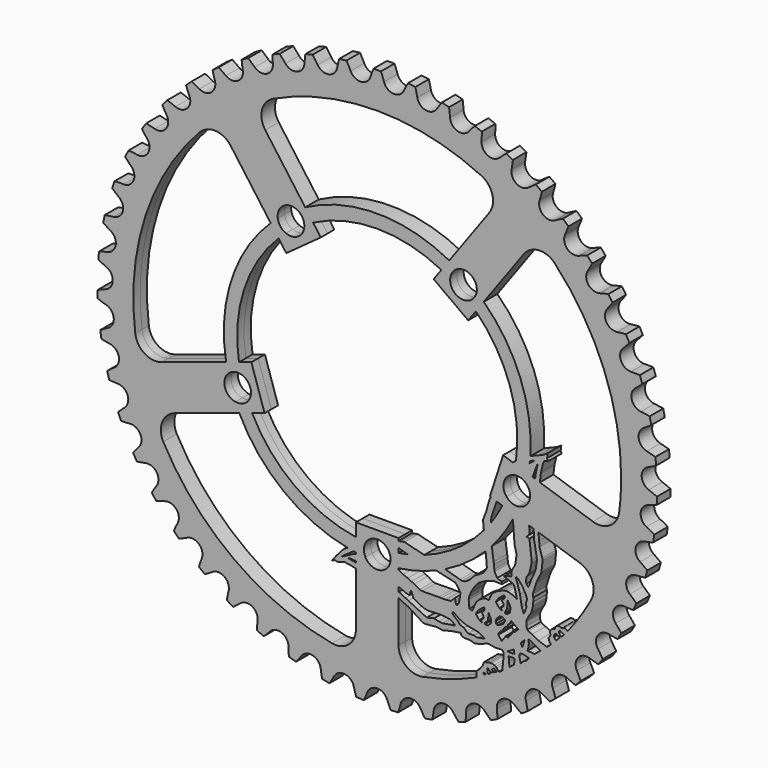
from build123d import *

# Parameters (mm, degrees)
F0_R     = 95.23914061
F2_DEPTH = 3.175
F3_DEPTH = 3.175


# Not quite as in the source:
# - a length typed as a fraction of an inch, garbled in the dataset ("3 / 203.2 mm" for 3/8 in), is restored


with BuildPart() as f2:
    # F0 (on Front) → F2 (new body, symmetric)
    with BuildSketch(Plane.XZ):
        with BuildLine():
            ThreePointArc((1.3974512393, 104.8471286678), (0, 104.8564411939), (-1.3974512393, 104.8471286678))
            ThreePointArc((-1.3974512393, 104.8471286678), (-1.9989055088, 103.3019703404), (-2.5462079028, 101.7368116953))
            ThreePointArc((-2.5462079028, 101.7368116953), (-3.9052398194, 99.8191421504), (-6.1056801538, 98.9930146972))
            ThreePointArc((-6.1056801538, 98.9930146972), (-8.3909636625, 99.5424721739), (-9.9753539423, 101.2785976519))
            ThreePointArc((-9.9753539423, 101.2785976519), (-10.7108477336, 102.7646361365), (-11.4976251519, 104.2241712642))
            ThreePointArc((-11.4976251519, 104.2241712642), (-12.8856288235, 104.061682812), (-14.2713436942, 103.880710476))
            ThreePointArc((-14.2713436942, 103.880710476), (-14.6783573813, 102.2733519742), (-15.0291718315, 100.6527993782))
            ThreePointArc((-15.0291718315, 100.6527993782), (-16.1422438465, 98.5826556819), (-18.224484574, 97.4923815023))
            ThreePointArc((-18.224484574, 97.4923815023), (-20.5599686886, 97.7568397874), (-22.34569959, 99.2851033058))
            ThreePointArc((-22.34569959, 99.2851033058), (-23.2582354424, 100.6694948013), (-24.2184092659, 102.0212816645))
            ThreePointArc((-24.2184092659, 102.0212816645), (-25.5759246489, 101.6894553933), (-26.9288971262, 101.3395666036))
            ThreePointArc((-26.9288971262, 101.3395666036), (-27.1353003181, 99.6943738437), (-27.2843088352, 98.0429932223))
            ThreePointArc((-27.2843088352, 98.0429932223), (-28.1345479113, 95.8517566428), (-30.0670243851, 94.5138631821))
            ThreePointArc((-30.0670243851, 94.5138631821), (-32.417305547, 94.4893133574), (-34.3773072098, 95.7865479992))
            ThreePointArc((-34.3773072098, 95.7865479992), (-35.45305201, 97.0483065417), (-36.5720669823, 98.2718534296))
            ThreePointArc((-36.5720669823, 98.2718534296), (-37.8785155273, 97.7757194874), (-39.1782359275, 97.2622182014))
            ThreePointArc((-39.1782359275, 97.2622182014), (-39.1808997623, 95.6041306286), (-39.125843529, 93.9469552287))
            ThreePointArc((-39.125843529, 93.9469552287), (-39.7003609085, 91.667842679), (-41.4537787551, 90.1026110382))
            ThreePointArc((-41.4537787551, 90.1026110382), (-43.7832290977, 89.7894252541), (-45.8877898946, 90.8359662645))
            ThreePointArc((-45.8877898946, 90.8359662645), (-47.110436448, 91.9559648806), (-48.3713294427, 93.0327240695))
            ThreePointArc((-48.3713294427, 93.0327240695), (-49.6069067216, 92.3798033412), (-50.8336726082, 91.7104737148))
            ThreePointArc((-50.8336726082, 91.7104737148), (-50.632556705, 90.0646262467), (-50.3742703176, 88.4267771581))
            ThreePointArc((-50.3742703176, 88.4267771581), (-50.6643569028, 86.0943376612), (-52.2121360949, 84.3254951565))
            ThreePointArc((-52.2121360949, 84.3254951565), (-54.4854435255, 83.7284209902), (-56.70266046, 84.5084038742))
            ThreePointArc((-56.70266046, 84.5084038742), (-58.0536746912, 85.4696645266), (-59.4373318558, 86.3833134448))
            ThreePointArc((-59.4373318558, 86.3833134448), (-60.5833077764, 85.5835035431), (-61.7185226292, 84.7684919313))
            ThreePointArc((-61.7185226292, 84.7684919313), (-61.3166757, 83.1598339377), (-60.8590745169, 81.5661392831))
            ThreePointArc((-60.8590745169, 81.5661392831), (-60.8603328907, 79.2157302442), (-62.1790106736, 77.2700907249))
            ThreePointArc((-62.1790106736, 77.2700907249), (-64.3617141688, 76.3981792122), (-66.6579764924, 76.8997802243))
            ThreePointArc((-66.6579764924, 76.8997802243), (-68.1168784028, 77.6877311814), (-69.6023249051, 78.4244198426))
            ThreePointArc((-69.6023249051, 78.4244198426), (-70.6413276406, 77.4898450703), (-71.6677827595, 76.5415062183))
            ThreePointArc((-71.6677827595, 76.5415062183), (-71.0712963941, 74.9944233147), (-70.4213171828, 73.4690418805))
            ThreePointArc((-70.4213171828, 73.4690418805), (-70.1337282697, 71.1362931047), (-71.2033148323, 69.0433504827))
            ThreePointArc((-71.2033148323, 69.0433504827), (-73.2623268321, 67.9098189133), (-75.6028255485, 68.1254342936))
            ThreePointArc((-75.6028255485, 68.1254342936), (-77.1474996722, 68.7281310219), (-78.7122176575, 69.276691977))
            ThreePointArc((-78.7122176575, 69.276691977), (-79.6284969855, 68.221519535), (-80.5306323574, 67.1542292932))
            ThreePointArc((-80.5306323574, 67.1542292932), (-79.748548681, 65.6921736793), (-78.9160444638, 64.2582286932))
            ThreePointArc((-78.9160444638, 64.2582286932), (-78.3439678185, 61.9785022741), (-79.1482493188, 59.7699834261))
            ThreePointArc((-79.1482493188, 59.7699834261), (-81.0523573, 58.3920149832), (-83.4016128346, 58.3183762222))
            ThreePointArc((-83.4016128346, 58.3183762222), (-85.0086434865, 58.7266824538), (-86.628913425, 59.0788000779))
            ThreePointArc((-86.628913425, 59.0788000779), (-87.408579485, 57.9190253048), (-88.172719657, 56.7489627052))
            ThreePointArc((-88.172719657, 56.7489627052), (-87.2168942611, 55.3940976539), (-86.2144849533, 54.0733262601))
            ThreePointArc((-86.2144849533, 54.0733262601), (-85.3665926745, 51.8811805265), (-85.8933770249, 49.5905643469))
            ThreePointArc((-85.8933770249, 49.5905643469), (-87.6137166516, 47.9890476274), (-89.9361166851, 47.6272710137))
            ThreePointArc((-89.9361166851, 47.6272710137), (-91.5811429185, 47.8349972424), (-93.2324031697, 47.9853337911))
            ThreePointArc((-93.2324031697, 47.9853337911), (-93.8636370189, 46.7385376903), (-94.478198405, 45.4834396894))
            ThreePointArc((-94.478198405, 45.4834396894), (-93.3631206282, 44.2563035737), (-92.2060017332, 43.0687273203))
            ThreePointArc((-92.2060017332, 43.0687273203), (-91.0951470036, 40.9973929669), (-91.3364486902, 38.6594028621))
            ThreePointArc((-91.3364486902, 38.6594028621), (-92.8469413671, 36.858615227), (-95.1072806824, 36.2141849253))
            ThreePointArc((-95.1072806824, 36.2141849253), (-96.7653655766, 36.2181822331), (-98.4225847182, 36.1644587577))
            ThreePointArc((-98.4225847182, 36.1644587577), (-98.8958174949, 34.8495414871), (-99.351483971, 33.5284340911))
            ThreePointArc((-99.351483971, 33.5284340911), (-98.0940572557, 32.4476290436), (-96.7997695163, 31.4112503761))
            ThreePointArc((-96.7997695163, 31.4112503761), (-95.4427917614, 29.4921267203), (-95.3949528966, 27.1422042371))
            ThreePointArc((-95.3949528966, 27.1422042371), (-96.6727010946, 25.1694437913), (-98.8367152516, 24.252128708))
            ThreePointArc((-98.8367152516, 24.252128708), (-100.4827239298, 24.0523364999), (-102.1207802088, 23.7953673935))
            ThreePointArc((-102.1207802088, 23.7953673935), (-102.4288381865, 22.4322617587), (-102.7187023133, 21.065171609))
            ThreePointArc((-102.7187023133, 21.065171609), (-101.3379879668, 20.1470815326), (-99.9261514659, 19.2776108951))
            ThreePointArc((-99.9261514659, 19.2776108951), (-98.343621085, 17.5397898952), (-98.0073668573, 15.2135574631))
            ThreePointArc((-98.0073668573, 15.2135574631), (-99.0330012161, 13.0987292441), (-101.0678859662, 11.9224349409))
            ThreePointArc((-101.0678859662, 11.9224349409), (-102.6768666145, 11.5218818629), (-104.2709287676, 11.0655625153))
            ThreePointArc((-104.2709287676, 11.0655625153), (-104.4091421014, 9.6749318081), (-104.5288098342, 8.2825825979))
            ThreePointArc((-104.5288098342, 8.2825825979), (-103.0457380786, 7.5411248023), (-101.5377548183, 6.8517424834))
            ThreePointArc((-101.5377548183, 6.8517424834), (-99.753661359, 5.3215677344), (-99.1340890397, 3.0542886658))
            ThreePointArc((-99.1340890397, 3.0542886658), (-99.8920619879, 0.8294513136), (-101.7669705525, -0.5879907869))
            ThreePointArc((-101.7669705525, -0.5879907869), (-103.3145326645, -1.1832327583), (-104.8404363343, -1.831985011))
            ThreePointArc((-104.8404363343, -1.831985011), (-104.8067098509, -3.2290602466), (-104.7543671488, -4.6255619225))
            ThreePointArc((-104.7543671488, -4.6255619225), (-103.1914198401, -5.1791476929), (-101.6101493096, -5.67799136))
            ThreePointArc((-101.6101493096, -5.67799136), (-99.6515378101, -6.9773239687), (-98.758039484, -9.1512800343))
            ThreePointArc((-98.758039484, -9.1512800343), (-99.2368609244, -11.4524002533), (-100.9233716008, -13.0895031738))
            ThreePointArc((-100.9233716008, -13.0895031738), (-102.3860557123, -13.870410777), (-103.8206697546, -14.701761512))
            ThreePointArc((-103.8206697546, -14.701761512), (-103.6155147131, -16.0841030394), (-103.3919550381, -17.4635876392))
            ThreePointArc((-103.3919550381, -17.4635876392), (-101.7728248644, -17.8209095885), (-100.142237513, -18.1216526423))
            ThreePointArc((-100.142237513, -18.1216526423), (-98.0387985272, -19.1704465528), (-96.8849187181, -21.2181246574))
            ThreePointArc((-96.8849187181, -21.2181246574), (-97.0773302057, -23.5606451062), (-98.5498772112, -25.3925920352))
            ThreePointArc((-98.5498772112, -25.3925920352), (-99.9055105221, -26.3473275071), (-101.2270876503, -27.3486742946))
            ThreePointArc((-101.2270876503, -27.3486742946), (-100.8536139921, -28.6953272254), (-100.4622262811, -30.0368831687))
            ThreePointArc((-100.4622262811, -30.0368831687), (-98.8114576053, -30.1925246603), (-97.1562714752, -30.2906081427))
            ThreePointArc((-97.1562714752, -30.2906081427), (-94.9398909938, -31.0729647084), (-93.5431213435, -32.9633241392))
            ThreePointArc((-93.5431213435, -32.9633241392), (-93.4462061162, -35.3117345958), (-94.6824671393, -37.3107550852))
            ThreePointArc((-94.6824671393, -37.3107550852), (-95.9104996304, -38.4248456091), (-97.0990060825, -39.5810090527))
            ThreePointArc((-97.0990060825, -39.5810090527), (-96.5628752875, -40.8715595011), (-96.0095925791, -42.1548501673))
            ThreePointArc((-96.0095925791, -42.1548501673), (-94.3522093717, -42.1064518349), (-92.6975153974, -42.0003889001))
            ThreePointArc((-92.6975153974, -42.0003889001), (-90.4017914894, -42.504448393), (-88.7833056019, -44.2088332281))
            ThreePointArc((-88.7833056019, -44.2088332281), (-88.3985327959, -46.5275341837), (-89.3797673795, -48.6633251205))
            ThreePointArc((-89.3797673795, -48.6633251205), (-90.4615833302, -49.9198822198), (-91.4990025598, -51.2133360601))
            ThreePointArc((-91.4990025598, -51.2133360601), (-90.8083418243, -52.4282205969), (-90.1015513205, -53.6337926077))
            ThreePointArc((-90.1015513205, -53.6337926077), (-88.4626778214, -53.3820881206), (-86.8335594768, -53.0734865747))
            ThreePointArc((-86.8335594768, -53.0734865747), (-84.4932929765, -53.2916079667), (-82.6776254481, -54.7841814692))
            ThreePointArc((-82.6776254481, -54.7841814692), (-82.0108278269, -57.0380237809), (-82.722161455, -59.2782087517))
            ThreePointArc((-82.722161455, -59.2782087517), (-83.6413616381, -60.6581843016), (-84.5119674272, -62.0693210969))
            ThreePointArc((-84.5119674272, -62.0693210969), (-83.677246464, -63.1901233109), (-82.8276623883, -64.2997014234))
            ThreePointArc((-82.8276623883, -64.2997014234), (-81.2321422492, -63.8485063651), (-79.6532953078, -63.342044293))
            ThreePointArc((-79.6532953078, -63.342044293), (-77.3039622698, -63.270921086), (-75.3186367695, -64.5290573631))
            ThreePointArc((-75.3186367695, -64.5290573631), (-74.3799223052, -66.683875079), (-74.8105718852, -68.9944951631))
            ThreePointArc((-74.8105718852, -68.9944951631), (-75.5532221629, -70.476970141), (-76.2438170152, -71.9843984958))
            ThreePointArc((-76.2438170152, -71.9843984958), (-75.2776893432, -72.9941281679), (-74.2981905242, -73.990892309))
            ThreePointArc((-74.2981905242, -73.990892309), (-72.770210204, -73.3470463367), (-71.265568376, -72.6504011871))
            ThreePointArc((-71.265568376, -72.6504011871), (-68.9427822944, -72.2911115366), (-66.817894333, -73.2957385248))
            ThreePointArc((-66.817894333, -73.2957385248), (-65.6214929802, -75.3188668047), (-65.7649303033, -77.664895357))
            ThreePointArc((-65.7649303033, -77.664895357), (-66.3197728544, -79.2273969532), (-66.8198880558, -80.8082657904))
            ThreePointArc((-66.8198880558, -80.8082657904), (-65.7369991858, -81.691616448), (-64.6424338271, -82.5604566893))
            ThreePointArc((-64.6424338271, -82.5604566893), (-63.20515595, -81.7337198516), (-61.7975280718, -80.857452055))
            ThreePointArc((-61.7975280718, -80.857452055), (-59.5365000158, -80.2154424257), (-57.3042607288, -80.9513310039))
            ThreePointArc((-57.3042607288, -80.9513310039), (-55.8683087124, -82.8121012854), (-55.7223594151, -85.1579749044))
            ThreePointArc((-55.7223594151, -85.1579749044), (-56.0809833921, -86.7768171877), (-56.3830377061, -88.407162147))
            ThreePointArc((-56.3830377061, -88.407162147), (-55.1998031293, -89.1507430946), (-54.006763726, -89.8784887038))
            ThreePointArc((-54.006763726, -89.8784887038), (-52.6819759595, -88.8813934884), (-51.3927002349, -87.8387863712))
            ThreePointArc((-51.3927002349, -87.8387863712), (-49.2277050852, -86.9237889748), (-46.9219529448, -87.3797838223))
            ThreePointArc((-46.9219529448, -87.3797838223), (-45.2682178335, -89.0499887246), (-44.8350943583, -91.3601463576))
            ThreePointArc((-44.8350943583, -91.3601463576), (-44.9920633874, -93.0107893289), (-45.0914779783, -94.6658960427))
            ThreePointArc((-45.0914779783, -94.6658960427), (-43.825834325, -95.2584353512), (-42.5524061384, -95.8340544466))
            ThreePointArc((-42.5524061384, -95.8340544466), (-41.3601909146, -94.6817158006), (-40.2088114494, -93.488574224))
            ThreePointArc((-40.2088114494, -93.488574224), (-38.1726683254, -92.3144594882), (-35.8283561837, -92.483648188))
            ThreePointArc((-35.8283561837, -92.483648188), (-33.9819069162, -93.9379691074), (-33.2681749735, -96.1773911194))
            ThreePointArc((-33.2681749735, -96.1773911194), (-33.2211095641, -97.834812714), (-33.1163774082, -99.4895914516))
            ThreePointArc((-33.1163774082, -99.4895914516), (-31.7875105459, -99.9221068289), (-30.4529974492, -100.3368736118))
            ThreePointArc((-30.4529974492, -100.3368736118), (-29.4114275356, -99.0467598146), (-28.4153980688, -97.7211705886))
            ThreePointArc((-28.4153980688, -97.7211705886), (-26.5389728249, -96.305736896), (-24.1916380643, -96.1855547198))
            ThreePointArc((-24.1916380643, -96.1855547198), (-22.1804649293, -97.4019456336), (-21.1969439678, -99.5366846697))
            ThreePointArc((-21.1969439678, -99.5366846697), (-20.9465575835, -101.1757600656), (-20.6392663135, -102.8051260681))
            ThreePointArc((-20.6392663135, -102.8051260681), (-19.2673205093, -103.0710610221), (-17.8919523608, -103.3186880509))
            ThreePointArc((-17.8919523608, -103.3186880509), (-17.0168168956, -101.9103559124), (-16.1912362186, -100.4724136185))
            ThreePointArc((-16.1912362186, -100.4724136185), (-14.5029735487, -98.8371175011), (-12.1881993714, -98.4293862882))
            ThreePointArc((-12.1881993714, -98.4293862882), (-10.0427897036, -99.38940795), (-8.8043888985, -101.3871035425))
            ThreePointArc((-8.8043888985, -101.3871035425), (-8.3544771417, -102.9829860275), (-7.84928498, -104.5622397672))
            ThreePointArc((-7.84928498, -104.5622397672), (-6.4550575339, -104.6575629951), (-5.0596835126, -104.7342964964))
            ThreePointArc((-5.0596835126, -104.7342964964), (-4.3642486574, -103.2290948963), (-3.7216317317, -101.7005972739))
            ThreePointArc((-3.7216317317, -101.7005972739), (-2.247123977, -99.8702281539), (0, -99.1811286939))
            ThreePointArc((0, -99.1811286939), (2.247123977, -99.8702281539), (3.7216317317, -101.7005972739))
            ThreePointArc((3.7216317317, -101.7005972739), (4.3642486574, -103.2290948963), (5.0596835126, -104.7342964964))
            ThreePointArc((5.0596835126, -104.7342964964), (6.4550575339, -104.6575629951), (7.84928498, -104.5622397672))
            ThreePointArc((7.84928498, -104.5622397672), (8.3544771417, -102.9829860275), (8.8043888985, -101.3871035425))
            ThreePointArc((8.8043888985, -101.3871035425), (10.0427897036, -99.38940795), (12.1881993714, -98.4293862882))
            ThreePointArc((12.1881993714, -98.4293862882), (14.5029735487, -98.8371175011), (16.1912362186, -100.4724136185))
            ThreePointArc((16.1912362186, -100.4724136185), (17.0168168956, -101.9103559124), (17.8919523608, -103.3186880509))
            ThreePointArc((17.8919523608, -103.3186880509), (19.2673205093, -103.0710610221), (20.6392663135, -102.8051260681))
            ThreePointArc((20.6392663135, -102.8051260681), (20.9465575835, -101.1757600656), (21.1969439678, -99.5366846697))
            ThreePointArc((21.1969439678, -99.5366846697), (22.1804649293, -97.4019456336), (24.1916380643, -96.1855547198))
            ThreePointArc((24.1916380643, -96.1855547198), (26.5389728249, -96.305736896), (28.4153980688, -97.7211705886))
            ThreePointArc((28.4153980688, -97.7211705886), (29.4114275356, -99.0467598146), (30.4529974492, -100.3368736118))
            ThreePointArc((30.4529974492, -100.3368736118), (31.7875105459, -99.9221068289), (33.1163774082, -99.4895914516))
            ThreePointArc((33.1163774082, -99.4895914516), (33.2211095641, -97.834812714), (33.2681749735, -96.1773911194))
            ThreePointArc((33.2681749735, -96.1773911194), (33.9819069162, -93.9379691074), (35.8283561837, -92.483648188))
            ThreePointArc((35.8283561837, -92.483648188), (38.1726683254, -92.3144594882), (40.2088114494, -93.488574224))
            ThreePointArc((40.2088114494, -93.488574224), (41.3601909146, -94.6817158006), (42.5524061384, -95.8340544466))
            ThreePointArc((42.5524061384, -95.8340544466), (43.825834325, -95.2584353512), (45.0914779783, -94.6658960427))
            ThreePointArc((45.0914779783, -94.6658960427), (44.9920633874, -93.0107893289), (44.8350943583, -91.3601463576))
            ThreePointArc((44.8350943583, -91.3601463576), (45.2682178335, -89.0499887246), (46.9219529448, -87.3797838223))
            ThreePointArc((46.9219529448, -87.3797838223), (49.2277050852, -86.9237889748), (51.3927002349, -87.8387863712))
            ThreePointArc((51.3927002349, -87.8387863712), (52.6819759595, -88.8813934884), (54.006763726, -89.8784887038))
            ThreePointArc((54.006763726, -89.8784887038), (55.1998031293, -89.1507430946), (56.3830377061, -88.407162147))
            ThreePointArc((56.3830377061, -88.407162147), (56.0809833921, -86.7768171877), (55.7223594151, -85.1579749044))
            ThreePointArc((55.7223594151, -85.1579749044), (55.8683087124, -82.8121012854), (57.3042607288, -80.9513310039))
            ThreePointArc((57.3042607288, -80.9513310039), (59.5365000158, -80.2154424257), (61.7975280718, -80.857452055))
            ThreePointArc((61.7975280718, -80.857452055), (63.20515595, -81.7337198516), (64.6424338271, -82.5604566893))
            ThreePointArc((64.6424338271, -82.5604566893), (65.7369991858, -81.691616448), (66.8198880558, -80.8082657904))
            ThreePointArc((66.8198880558, -80.8082657904), (66.3197728544, -79.2273969532), (65.7649303033, -77.664895357))
            ThreePointArc((65.7649303033, -77.664895357), (65.6214929802, -75.3188668047), (66.817894333, -73.2957385248))
            ThreePointArc((66.817894333, -73.2957385248), (68.9427822944, -72.2911115366), (71.265568376, -72.6504011871))
            ThreePointArc((71.265568376, -72.6504011871), (72.770210204, -73.3470463367), (74.2981905242, -73.990892309))
            ThreePointArc((74.2981905242, -73.990892309), (75.2776893432, -72.9941281679), (76.2438170152, -71.9843984958))
            ThreePointArc((76.2438170152, -71.9843984958), (75.5532221629, -70.476970141), (74.8105718852, -68.9944951631))
            ThreePointArc((74.8105718852, -68.9944951631), (74.3799223052, -66.683875079), (75.3186367695, -64.5290573631))
            ThreePointArc((75.3186367695, -64.5290573631), (77.3039622698, -63.270921086), (79.6532953078, -63.342044293))
            ThreePointArc((79.6532953078, -63.342044293), (81.2321422492, -63.8485063651), (82.8276623883, -64.2997014234))
            ThreePointArc((82.8276623883, -64.2997014234), (83.677246464, -63.1901233109), (84.5119674272, -62.0693210969))
            ThreePointArc((84.5119674272, -62.0693210969), (83.6413616381, -60.6581843016), (82.722161455, -59.2782087517))
            ThreePointArc((82.722161455, -59.2782087517), (82.0108278269, -57.0380237809), (82.6776254481, -54.7841814692))
            ThreePointArc((82.6776254481, -54.7841814692), (84.4932929765, -53.2916079667), (86.8335594768, -53.0734865747))
            ThreePointArc((86.8335594768, -53.0734865747), (88.4626778214, -53.3820881206), (90.1015513205, -53.6337926077))
            ThreePointArc((90.1015513205, -53.6337926077), (90.8083418243, -52.4282205969), (91.4990025598, -51.2133360601))
            ThreePointArc((91.4990025598, -51.2133360601), (90.4615833302, -49.9198822198), (89.3797673795, -48.6633251205))
            ThreePointArc((89.3797673795, -48.6633251205), (88.3985327959, -46.5275341837), (88.7833056019, -44.2088332281))
            ThreePointArc((88.7833056019, -44.2088332281), (90.4017914894, -42.504448393), (92.6975153974, -42.0003889001))
            ThreePointArc((92.6975153974, -42.0003889001), (94.3522093717, -42.1064518349), (96.0095925791, -42.1548501673))
            ThreePointArc((96.0095925791, -42.1548501673), (96.5628752875, -40.8715595011), (97.0990060825, -39.5810090527))
            ThreePointArc((97.0990060825, -39.5810090527), (95.9104996304, -38.4248456091), (94.6824671393, -37.3107550852))
            ThreePointArc((94.6824671393, -37.3107550852), (93.4462061162, -35.3117345958), (93.5431213435, -32.9633241392))
            ThreePointArc((93.5431213435, -32.9633241392), (94.9398909938, -31.0729647084), (97.1562714752, -30.2906081427))
            ThreePointArc((97.1562714752, -30.2906081427), (98.8114576053, -30.1925246603), (100.4622262811, -30.0368831687))
            ThreePointArc((100.4622262811, -30.0368831687), (100.8536139921, -28.6953272254), (101.2270876503, -27.3486742946))
            ThreePointArc((101.2270876503, -27.3486742946), (99.9055105221, -26.3473275071), (98.5498772112, -25.3925920352))
            ThreePointArc((98.5498772112, -25.3925920352), (97.0773302057, -23.5606451062), (96.8849187181, -21.2181246574))
            ThreePointArc((96.8849187181, -21.2181246574), (98.0387985272, -19.1704465528), (100.142237513, -18.1216526423))
            ThreePointArc((100.142237513, -18.1216526423), (101.7728248644, -17.8209095885), (103.3919550381, -17.4635876392))
            ThreePointArc((103.3919550381, -17.4635876392), (103.6155147131, -16.0841030394), (103.8206697546, -14.701761512))
            ThreePointArc((103.8206697546, -14.701761512), (102.3860557123, -13.870410777), (100.9233716008, -13.0895031738))
            ThreePointArc((100.9233716008, -13.0895031738), (99.2368609244, -11.4524002533), (98.758039484, -9.1512800343))
            ThreePointArc((98.758039484, -9.1512800343), (99.6515378101, -6.9773239687), (101.6101493096, -5.67799136))
            ThreePointArc((101.6101493096, -5.67799136), (103.1914198401, -5.1791476929), (104.7543671488, -4.6255619225))
            ThreePointArc((104.7543671488, -4.6255619225), (104.8067098509, -3.2290602466), (104.8404363343, -1.831985011))
            ThreePointArc((104.8404363343, -1.831985011), (103.3145326645, -1.1832327583), (101.7669705525, -0.5879907869))
            ThreePointArc((101.7669705525, -0.5879907869), (99.8920619879, 0.8294513136), (99.1340890397, 3.0542886658))
            ThreePointArc((99.1340890397, 3.0542886658), (99.753661359, 5.3215677344), (101.5377548183, 6.8517424834))
            ThreePointArc((101.5377548183, 6.8517424834), (103.0457380786, 7.5411248023), (104.5288098342, 8.2825825979))
            ThreePointArc((104.5288098342, 8.2825825979), (104.4091421014, 9.6749318081), (104.2709287676, 11.0655625153))
            ThreePointArc((104.2709287676, 11.0655625153), (102.6768666145, 11.5218818629), (101.0678859662, 11.9224349409))
            ThreePointArc((101.0678859662, 11.9224349409), (99.0330012161, 13.0987292441), (98.0073668573, 15.2135574631))
            ThreePointArc((98.0073668573, 15.2135574631), (98.343621085, 17.5397898952), (99.9261514659, 19.2776108951))
            ThreePointArc((99.9261514659, 19.2776108951), (101.3379879668, 20.1470815326), (102.7187023133, 21.065171609))
            ThreePointArc((102.7187023133, 21.065171609), (102.4288381865, 22.4322617587), (102.1207802088, 23.7953673935))
            ThreePointArc((102.1207802088, 23.7953673935), (100.4827239298, 24.0523364999), (98.8367152516, 24.252128708))
            ThreePointArc((98.8367152516, 24.252128708), (96.6727010946, 25.1694437913), (95.3949528966, 27.1422042371))
            ThreePointArc((95.3949528966, 27.1422042371), (95.4427917614, 29.4921267203), (96.7997695163, 31.4112503761))
            ThreePointArc((96.7997695163, 31.4112503761), (98.0940572557, 32.4476290436), (99.351483971, 33.5284340911))
            ThreePointArc((99.351483971, 33.5284340911), (98.8958174949, 34.8495414871), (98.4225847182, 36.1644587577))
            ThreePointArc((98.4225847182, 36.1644587577), (96.7653655766, 36.2181822331), (95.1072806824, 36.2141849253))
            ThreePointArc((95.1072806824, 36.2141849253), (92.8469413671, 36.858615227), (91.3364486902, 38.6594028621))
            ThreePointArc((91.3364486902, 38.6594028621), (91.0951470036, 40.9973929669), (92.2060017332, 43.0687273203))
            ThreePointArc((92.2060017332, 43.0687273203), (93.3631206282, 44.2563035737), (94.478198405, 45.4834396894))
            ThreePointArc((94.478198405, 45.4834396894), (93.8636370189, 46.7385376903), (93.2324031697, 47.9853337911))
            ThreePointArc((93.2324031697, 47.9853337911), (91.5811429185, 47.8349972424), (89.9361166851, 47.6272710137))
            ThreePointArc((89.9361166851, 47.6272710137), (87.6137166516, 47.9890476274), (85.8933770249, 49.5905643469))
            ThreePointArc((85.8933770249, 49.5905643469), (85.3665926745, 51.8811805265), (86.2144849533, 54.0733262601))
            ThreePointArc((86.2144849533, 54.0733262601), (87.2168942611, 55.3940976539), (88.172719657, 56.7489627052))
            ThreePointArc((88.172719657, 56.7489627052), (87.408579485, 57.9190253048), (86.628913425, 59.0788000779))
            ThreePointArc((86.628913425, 59.0788000779), (85.0086434865, 58.7266824538), (83.4016128346, 58.3183762222))
            ThreePointArc((83.4016128346, 58.3183762222), (81.0523573, 58.3920149832), (79.1482493188, 59.7699834261))
            ThreePointArc((79.1482493188, 59.7699834261), (78.3439678185, 61.9785022741), (78.9160444638, 64.2582286932))
            ThreePointArc((78.9160444638, 64.2582286932), (79.748548681, 65.6921736793), (80.5306323574, 67.1542292932))
            ThreePointArc((80.5306323574, 67.1542292932), (79.6284969855, 68.221519535), (78.7122176575, 69.276691977))
            ThreePointArc((78.7122176575, 69.276691977), (77.1474996722, 68.7281310219), (75.6028255485, 68.1254342936))
            ThreePointArc((75.6028255485, 68.1254342936), (73.2623268321, 67.9098189133), (71.2033148323, 69.0433504827))
            ThreePointArc((71.2033148323, 69.0433504827), (70.1337282697, 71.1362931047), (70.4213171828, 73.4690418805))
            ThreePointArc((70.4213171828, 73.4690418805), (71.0712963941, 74.9944233147), (71.6677827595, 76.5415062183))
            ThreePointArc((71.6677827595, 76.5415062183), (70.6413276406, 77.4898450703), (69.6023249051, 78.4244198426))
            ThreePointArc((69.6023249051, 78.4244198426), (68.1168784028, 77.6877311814), (66.6579764924, 76.8997802243))
            ThreePointArc((66.6579764924, 76.8997802243), (64.3617141688, 76.3981792122), (62.1790106736, 77.2700907249))
            ThreePointArc((62.1790106736, 77.2700907249), (60.8603328907, 79.2157302442), (60.8590745169, 81.5661392831))
            ThreePointArc((60.8590745169, 81.5661392831), (61.3166757, 83.1598339377), (61.7185226292, 84.7684919313))
            ThreePointArc((61.7185226292, 84.7684919313), (60.5833077764, 85.5835035431), (59.4373318558, 86.3833134448))
            ThreePointArc((59.4373318558, 86.3833134448), (58.0536746912, 85.4696645266), (56.70266046, 84.5084038742))
            ThreePointArc((56.70266046, 84.5084038742), (54.4854435255, 83.7284209902), (52.2121360949, 84.3254951565))
            ThreePointArc((52.2121360949, 84.3254951565), (50.6643569028, 86.0943376612), (50.3742703176, 88.4267771581))
            ThreePointArc((50.3742703176, 88.4267771581), (50.632556705, 90.0646262467), (50.8336726082, 91.7104737148))
            ThreePointArc((50.8336726082, 91.7104737148), (49.6069067216, 92.3798033412), (48.3713294427, 93.0327240695))
            ThreePointArc((48.3713294427, 93.0327240695), (47.110436448, 91.9559648806), (45.8877898946, 90.8359662645))
            ThreePointArc((45.8877898946, 90.8359662645), (43.7832290977, 89.7894252541), (41.4537787551, 90.1026110382))
            ThreePointArc((41.4537787551, 90.1026110382), (39.7003609085, 91.667842679), (39.125843529, 93.9469552287))
            ThreePointArc((39.125843529, 93.9469552287), (39.1808997623, 95.6041306286), (39.1782359275, 97.2622182014))
            ThreePointArc((39.1782359275, 97.2622182014), (37.8785155273, 97.7757194874), (36.5720669823, 98.2718534296))
            ThreePointArc((36.5720669823, 98.2718534296), (35.45305201, 97.0483065417), (34.3773072098, 95.7865479992))
            ThreePointArc((34.3773072098, 95.7865479992), (32.417305547, 94.4893133574), (30.0670243851, 94.5138631821))
            ThreePointArc((30.0670243851, 94.5138631821), (28.1345479113, 95.8517566428), (27.2843088352, 98.0429932223))
            ThreePointArc((27.2843088352, 98.0429932223), (27.1353003181, 99.6943738437), (26.9288971262, 101.3395666036))
            ThreePointArc((26.9288971262, 101.3395666036), (25.5759246489, 101.6894553933), (24.2184092659, 102.0212816645))
            ThreePointArc((24.2184092659, 102.0212816645), (23.2582354424, 100.6694948013), (22.34569959, 99.2851033058))
            ThreePointArc((22.34569959, 99.2851033058), (20.5599686886, 97.7568397874), (18.224484574, 97.4923815023))
            ThreePointArc((18.224484574, 97.4923815023), (16.1422438465, 98.5826556819), (15.0291718315, 100.6527993782))
            ThreePointArc((15.0291718315, 100.6527993782), (14.6783573813, 102.2733519742), (14.2713436942, 103.880710476))
            ThreePointArc((14.2713436942, 103.880710476), (12.8856288235, 104.061682812), (11.4976251519, 104.2241712642))
            ThreePointArc((11.4976251519, 104.2241712642), (10.7108477336, 102.7646361365), (9.9753539423, 101.2785976519))
            ThreePointArc((9.9753539423, 101.2785976519), (8.3909636625, 99.5424721739), (6.1056801538, 98.9930146972))
            ThreePointArc((6.1056801538, 98.9930146972), (3.9052398194, 99.8191421504), (2.5462079028, 101.7368116953))
            ThreePointArc((2.5462079028, 101.7368116953), (1.9989055088, 103.3019703404), (1.3974512393, 104.8471286678))
        make_face()
        Circle(F0_R, mode=Mode.SUBTRACT)
        Circle(F0_R)
        with BuildLine():
            ThreePointArc((80.1881548429, -43.922062515), (53.7407004803, -73.9677285346), (16.99286117, -89.8361309382))
            ThreePointArc((16.99286117, -89.8361309382), (0, -91.42914061), (-16.99286117, -89.8361309382))
            ThreePointArc((-16.99286117, -89.8361309382), (-53.7407004803, -73.9677285346), (-80.1881548429, -43.922062515))
            ThreePointArc((-80.1881548429, -43.922062515), (-86.9542799564, -28.2531582296), (-90.6903206121, -11.5997198226))
            ThreePointArc((-90.6903206121, -11.5997198226), (-86.9542799564, 28.2531582296), (-66.551866358, 62.6908034479))
            ThreePointArc((-66.551866358, 62.6908034479), (-53.7407004803, 73.9677285346), (-39.0568394189, 82.6671098278))
            ThreePointArc((-39.0568394189, 82.6671098278), (0, 91.42914061), (39.0568394189, 82.6671098278))
            ThreePointArc((39.0568394189, 82.6671098278), (53.7407004803, 73.9677285346), (66.551866358, 62.6908034479))
            ThreePointArc((66.551866358, 62.6908034479), (84.9825502671, 33.7231953229), (91.42914061, 0))
            ThreePointArc((91.42914061, 0), (91.2442486623, -5.8116124043), (90.6903206121, -11.5997198226))
            ThreePointArc((90.6903206121, -11.5997198226), (86.9542799564, -28.2531582296), (80.1881548429, -43.922062515))
        make_face(mode=Mode.SUBTRACT)
        with BuildLine():
            ThreePointArc((-39.0568394189, 82.6671098278), (-53.7407004803, 73.9677285346), (-66.551866358, 62.6908034479))
            ThreePointArc((-66.551866358, 62.6908034479), (-60.5498122767, 65.0591158248), (-54.8967300593, 61.9484538129))
            Line((-54.8967300593, 61.9484538129), (-39.9410741663, 41.3637594331))
            ThreePointArc((-39.9410741663, 41.3637594331), (-38.6277782996, 42.592778069), (-37.2766843665, 43.7801188057))
            ThreePointArc((-37.2766843665, 43.7801188057), (-35.2671151375, 48.5410196625), (-30.1182383111, 48.9810342994))
            ThreePointArc((-30.1182383111, 48.9810342994), (-28.5714991801, 49.8990925228), (-26.9968022563, 50.7683234698))
            Line((-26.9968022563, 50.7683234698), (-41.9524581493, 71.3530178496))
            ThreePointArc((-41.9524581493, 71.3530178496), (-43.1639750498, 77.6906659551), (-39.0568394189, 82.6671098278))
        make_face()
        with BuildLine():
            ThreePointArc((37.2766843665, 43.7801188057), (38.6277782996, 42.592778069), (39.9410741663, 41.3637594331))
            Line((39.9410741663, 41.3637594331), (54.8967300593, 61.9484538129))
            ThreePointArc((54.8967300593, 61.9484538129), (60.5498122767, 65.0591158248), (66.551866358, 62.6908034479))
            ThreePointArc((66.551866358, 62.6908034479), (53.7407004803, 73.9677285346), (39.0568394189, 82.6671098278))
            ThreePointArc((39.0568394189, 82.6671098278), (43.1639750498, 77.6906659551), (41.9524581493, 71.3530178496))
            Line((41.9524581493, 71.3530178496), (26.9968022563, 50.7683234698))
            ThreePointArc((26.9968022563, 50.7683234698), (28.5714991801, 49.8990925228), (30.1182383111, 48.9810342994))
            ThreePointArc((30.1182383111, 48.9810342994), (34.9692348029, 48.7415060788), (37.3281888761, 44.4959346906))
            ThreePointArc((37.3281888761, 44.4959346906), (37.3152961264, 44.1371014788), (37.2766843665, 43.7801188057))
        make_face()
        with BuildLine():
            ThreePointArc((53.1564962375, -21.923432846), (52.4447790792, -23.5753080009), (51.6817436383, -25.2041142377))
            Line((51.6817436383, -25.2041142377), (75.8805031971, -33.0667678427))
            ThreePointArc((75.8805031971, -33.0667678427), (80.5858170493, -37.4819210974), (80.1881548429, -43.922062515))
            ThreePointArc((80.1881548429, -43.922062515), (86.9542799564, -28.2531582296), (90.6903206121, -11.5997198226))
            ThreePointArc((90.6903206121, -11.5997198226), (87.2266159471, -17.0436436559), (80.8247751071, -17.849863582))
            Line((80.8247751071, -17.849863582), (56.6260155483, -9.9872099769))
            ThreePointArc((56.6260155483, -9.9872099769), (56.2859359025, -11.7534428821), (55.8907793241, -13.5081748045))
            ThreePointArc((55.8907793241, -13.5081748045), (56.9402436835, -15.1135631331), (57.3081083962, -16.9959346906))
            ThreePointArc((57.3081083962, -16.9959346906), (56.1318460446, -20.2175849505), (53.1564962375, -21.923432846))
        make_face()
        with BuildLine():
            Line((-75.8805031971, -33.0667678427), (-51.6817436383, -25.2041142377))
            ThreePointArc((-51.6817436383, -25.2041142377), (-52.4447790792, -23.5753080009), (-53.1564962375, -21.923432846))
            ThreePointArc((-53.1564962375, -21.923432846), (-57.0633909777, -18.5410196625), (-55.8907793241, -13.5081748045))
            ThreePointArc((-55.8907793241, -13.5081748045), (-56.2859359025, -11.7534428821), (-56.6260155483, -9.9872099769))
            Line((-56.6260155483, -9.9872099769), (-80.8247751071, -17.849863582))
            ThreePointArc((-80.8247751071, -17.849863582), (-87.2266159471, -17.0436436559), (-90.6903206121, -11.5997198226))
            ThreePointArc((-90.6903206121, -11.5997198226), (-86.9542799564, -28.2531582296), (-80.1881548429, -43.922062515))
            ThreePointArc((-80.1881548429, -43.922062515), (-80.5858170493, -37.4819210974), (-75.8805031971, -33.0667678427))
        make_face()
        with BuildLine():
            ThreePointArc((8, -56.9407586883), (6.2151222962, -57.1631197088), (4.4241629689, -57.3295454545))
            ThreePointArc((4.4241629689, -57.3295454545), (0, -60), (-4.4241629689, -57.3295454545))
            ThreePointArc((-4.4241629689, -57.3295454545), (-6.2151222962, -57.1631197088), (-8, -56.9407586883))
            Line((-8, -56.9407586883), (-8, -82.3848402378))
            ThreePointArc((-8, -82.3848402378), (-10.7450383291, -88.2242170266), (-16.99286117, -89.8361309382))
            ThreePointArc((-16.99286117, -89.8361309382), (0, -91.42914061), (16.99286117, -89.8361309382))
            ThreePointArc((16.99286117, -89.8361309382), (10.7450383291, -88.2242170266), (8, -82.3848402378))
            Line((8, -82.3848402378), (8, -56.9407586883))
        make_face()
        with BuildLine():
            Line((-8, -56.9407586883), (-8, -51.8868962263))
            ThreePointArc((-8, -51.8868962263), (-30.8587257454, -42.4733922047), (-46.8752348114, -23.6423848497))
            Line((-46.8752348114, -23.6423848497), (-51.6817436383, -25.2041142377))
            ThreePointArc((-51.6817436383, -25.2041142377), (-33.7976520068, -46.5184771766), (-8, -56.9407586883))
        make_face()
        with BuildLine():
            Line((-56.6260155483, -9.9872099769), (-51.8195067214, -8.4254805889))
            ThreePointArc((-51.8195067214, -8.4254805889), (-49.9304671055, 16.2233922047), (-36.9704883441, 37.2750988141))
            Line((-36.9704883441, 37.2750988141), (-39.9410741663, 41.3637594331))
            ThreePointArc((-39.9410741663, 41.3637594331), (-54.685749687, 17.7684771766), (-56.6260155483, -9.9872099769))
        make_face()
        with BuildLine():
            ThreePointArc((-24.0262164341, 46.6796628508), (0, 52.5), (24.0262164341, 46.6796628508))
            Line((24.0262164341, 46.6796628508), (26.9968022563, 50.7683234698))
            ThreePointArc((26.9968022563, 50.7683234698), (0, 57.5), (-26.9968022563, 50.7683234698))
            Line((-26.9968022563, 50.7683234698), (-24.0262164341, 46.6796628508))
        make_face()
        with BuildLine():
            ThreePointArc((36.9704883441, 37.2750988141), (49.9304671055, 16.2233922047), (51.8195067214, -8.4254805889))
            Line((51.8195067214, -8.4254805889), (56.6260155483, -9.9872099769))
            ThreePointArc((56.6260155483, -9.9872099769), (54.685749687, 17.7684771766), (39.9410741663, 41.3637594331))
            Line((39.9410741663, 41.3637594331), (36.9704883441, 37.2750988141))
        make_face()
        with BuildLine():
            ThreePointArc((46.8752348114, -23.6423848497), (30.8587257454, -42.4733922047), (8, -51.8868962263))
            Line((8, -51.8868962263), (8, -56.9407586883))
            ThreePointArc((8, -56.9407586883), (33.7976520068, -46.5184771766), (51.6817436383, -25.2041142377))
            Line((51.6817436383, -25.2041142377), (46.8752348114, -23.6423848497))
        make_face()
        with BuildLine():
            ThreePointArc((-4.2271352617, -52.3295454545), (0, -50), (4.2271352617, -52.3295454545))
            ThreePointArc((4.2271352617, -52.3295454545), (6.1175725383, -52.1423561631), (8, -51.8868962263))
            Line((8, -51.8868962263), (8, -47))
            Line((8, -47), (-8, -47))
            Line((-8, -47), (-8, -51.8868962263))
            ThreePointArc((-8, -51.8868962263), (-6.1175725383, -52.1423561631), (-4.2271352617, -52.3295454545))
        make_face()
        with BuildLine():
            Line((34.0980428127, 33.3215167173), (36.9704883441, 37.2750988141))
            ThreePointArc((36.9704883441, 37.2750988141), (35.5977281203, 38.5882333448), (34.1783593416, 39.8508438144))
            ThreePointArc((34.1783593416, 39.8508438144), (29.3892626146, 40.4508497187), (27.3387108131, 44.8201393469))
            ThreePointArc((27.3387108131, 44.8201393469), (25.6992878246, 45.7798711806), (24.0262164341, 46.6796628508))
            Line((24.0262164341, 46.6796628508), (21.1537709027, 42.726080754))
            Line((21.1537709027, 42.726080754), (34.0980428127, 33.3215167173))
        make_face()
        with BuildLine():
            ThreePointArc((-34.1783593416, 39.8508438144), (-35.5977281203, 38.5882333448), (-36.9704883441, 37.2750988141))
            Line((-36.9704883441, 37.2750988141), (-34.0980428127, 33.3215167173))
            Line((-34.0980428127, 33.3215167173), (-21.1537709027, 42.726080754))
            Line((-21.1537709027, 42.726080754), (-24.0262164341, 46.6796628508))
            ThreePointArc((-24.0262164341, 46.6796628508), (-25.6992878246, 45.7798711806), (-27.3387108131, 44.8201393469))
            ThreePointArc((-27.3387108131, 44.8201393469), (-27.3308200527, 44.6581223677), (-27.3281888761, 44.4959346906))
            ThreePointArc((-27.3281888761, 44.4959346906), (-29.5220217684, 40.3576468606), (-34.1783593416, 39.8508438144))
        make_face()
        with BuildLine():
            ThreePointArc((-48.4620985659, -20.1909633893), (-47.6998937252, -21.9310314076), (-46.8752348114, -23.6423848497))
            Line((-46.8752348114, -23.6423848497), (-42.2275203109, -22.132250866))
            Line((-42.2275203109, -22.132250866), (-47.1717922209, -6.9153466053))
            Line((-47.1717922209, -6.9153466053), (-51.8195067214, -8.4254805889))
            ThreePointArc((-51.8195067214, -8.4254805889), (-51.4807614826, -10.2947169547), (-51.0746118327, -12.1504743175))
            ThreePointArc((-51.0746118327, -12.1504743175), (-48.3604836156, -13.9273424089), (-47.3081083962, -16.9959346906))
            ThreePointArc((-47.3081083962, -16.9959346906), (-47.6054469609, -18.6944562313), (-48.4620985659, -20.1909633893))
        make_face()
        with BuildLine():
            Line((42.2275203109, -22.132250866), (46.8752348114, -23.6423848497))
            ThreePointArc((46.8752348114, -23.6423848497), (47.6998937252, -21.9310314076), (48.4620985659, -20.1909633893))
            ThreePointArc((48.4620985659, -20.1909633893), (47.5528258148, -15.4508497187), (51.0746118327, -12.1504743175))
            ThreePointArc((51.0746118327, -12.1504743175), (51.4807614826, -10.2947169547), (51.8195067214, -8.4254805889))
            Line((51.8195067214, -8.4254805889), (47.1717922209, -6.9153466053))
            Line((47.1717922209, -6.9153466053), (42.2275203109, -22.132250866))
        make_face()
        with BuildLine():
            ThreePointArc((34.1783593416, 39.8508438144), (35.5977281203, 38.5882333448), (36.9704883441, 37.2750988141))
            Line((36.9704883441, 37.2750988141), (39.9410741663, 41.3637594331))
            ThreePointArc((39.9410741663, 41.3637594331), (38.6277782996, 42.592778069), (37.2766843665, 43.7801188057))
            ThreePointArc((37.2766843665, 43.7801188057), (36.254416733, 41.4000124023), (34.1783593416, 39.8508438144))
        make_face()
        with BuildLine():
            ThreePointArc((24.0262164341, 46.6796628508), (25.6992878246, 45.7798711806), (27.3387108131, 44.8201393469))
            ThreePointArc((27.3387108131, 44.8201393469), (28.1705206782, 47.273306678), (30.1182383111, 48.9810342994))
            ThreePointArc((30.1182383111, 48.9810342994), (28.5714991801, 49.8990925228), (26.9968022563, 50.7683234698))
            Line((26.9968022563, 50.7683234698), (24.0262164341, 46.6796628508))
        make_face()
        with BuildLine():
            Line((-39.9410741663, 41.3637594331), (-36.9704883441, 37.2750988141))
            ThreePointArc((-36.9704883441, 37.2750988141), (-35.5977281203, 38.5882333448), (-34.1783593416, 39.8508438144))
            ThreePointArc((-34.1783593416, 39.8508438144), (-36.254416733, 41.4000124023), (-37.2766843665, 43.7801188057))
            ThreePointArc((-37.2766843665, 43.7801188057), (-38.6277782996, 42.592778069), (-39.9410741663, 41.3637594331))
        make_face()
        with BuildLine():
            ThreePointArc((-26.9968022563, 50.7683234698), (-28.5714991801, 49.8990925228), (-30.1182383111, 48.9810342994))
            ThreePointArc((-30.1182383111, 48.9810342994), (-28.1705206782, 47.273306678), (-27.3387108131, 44.8201393469))
            ThreePointArc((-27.3387108131, 44.8201393469), (-25.6992878246, 45.7798711806), (-24.0262164341, 46.6796628508))
            Line((-24.0262164341, 46.6796628508), (-26.9968022563, 50.7683234698))
        make_face()
        with BuildLine():
            ThreePointArc((-56.6260155483, -9.9872099769), (-56.2859359025, -11.7534428821), (-55.8907793241, -13.5081748045))
            ThreePointArc((-55.8907793241, -13.5081748045), (-53.6647559929, -12.1835021146), (-51.0746118327, -12.1504743175))
            ThreePointArc((-51.0746118327, -12.1504743175), (-51.4807614826, -10.2947169547), (-51.8195067214, -8.4254805889))
            Line((-51.8195067214, -8.4254805889), (-56.6260155483, -9.9872099769))
        make_face()
        with BuildLine():
            Line((-51.6817436383, -25.2041142377), (-46.8752348114, -23.6423848497))
            ThreePointArc((-46.8752348114, -23.6423848497), (-47.6998937252, -21.9310314076), (-48.4620985659, -20.1909633893))
            ThreePointArc((-48.4620985659, -20.1909633893), (-50.5769824615, -21.6866918788), (-53.1564962375, -21.923432846))
            ThreePointArc((-53.1564962375, -21.923432846), (-52.4447790792, -23.5753080009), (-51.6817436383, -25.2041142377))
        make_face()
        with BuildLine():
            ThreePointArc((-4.4241629689, -57.3295454545), (-4.9961225234, -54.8031250869), (-4.2271352617, -52.3295454545))
            ThreePointArc((-4.2271352617, -52.3295454545), (-6.1175725383, -52.1423561631), (-8, -51.8868962263))
            Line((-8, -51.8868962263), (-8, -56.9407586883))
            ThreePointArc((-8, -56.9407586883), (-6.2151222962, -57.1631197088), (-4.4241629689, -57.3295454545))
        make_face()
        with BuildLine():
            ThreePointArc((51.8195067214, -8.4254805889), (51.4807614826, -10.2947169547), (51.0746118327, -12.1504743175))
            ThreePointArc((51.0746118327, -12.1504743175), (53.6647559929, -12.1835021146), (55.8907793241, -13.5081748045))
            ThreePointArc((55.8907793241, -13.5081748045), (56.2859359025, -11.7534428821), (56.6260155483, -9.9872099769))
            Line((56.6260155483, -9.9872099769), (51.8195067214, -8.4254805889))
        make_face()
        with BuildLine():
            ThreePointArc((48.4620985659, -20.1909633893), (47.6998937252, -21.9310314076), (46.8752348114, -23.6423848497))
            Line((46.8752348114, -23.6423848497), (51.6817436383, -25.2041142377))
            ThreePointArc((51.6817436383, -25.2041142377), (52.4447790792, -23.5753080009), (53.1564962375, -21.923432846))
            ThreePointArc((53.1564962375, -21.923432846), (50.5769824615, -21.6866918788), (48.4620985659, -20.1909633893))
        make_face()
        with BuildLine():
            ThreePointArc((4.2271352617, -52.3295454545), (4.8028989323, -53.6099777535), (5, -55))
            ThreePointArc((5, -55), (4.8539064085, -56.1998302287), (4.4241629689, -57.3295454545))
            ThreePointArc((4.4241629689, -57.3295454545), (6.2151222962, -57.1631197088), (8, -56.9407586883))
            Line((8, -56.9407586883), (8, -51.8868962263))
            ThreePointArc((8, -51.8868962263), (6.1175725383, -52.1423561631), (4.2271352617, -52.3295454545))
        make_face()
    extrude(amount=F2_DEPTH, both=True)

    # F1 (on Front) → F3 (join, symmetric)
    with BuildSketch(Plane.XZ):
        with BuildLine():
            ThreePointArc((37.2109275745, -83.5142779513), (55.8993511569, -72.3501920725), (71.4188006216, -57.084522162))
            Line((71.4188006216, -57.084522162), (71.320169028, -57.0210753741))
            Line((71.320169028, -57.0210753741), (70.3312450591, -56.5019277754))
            Line((70.3312450591, -56.5019277754), (70.1337319623, -56.4765244414))
            Line((70.1337319623, -56.4765244414), (69.5419024751, -56.5190190124))
            Line((69.5419024751, -56.5190190124), (69.3658390843, -56.9077958996))
            Line((69.3658390843, -56.9077958996), (68.5796559745, -56.6095417739))
            Line((68.5796559745, -56.6095417739), (68.1365751235, -56.5255287159))
            Line((68.1365751235, -56.5255287159), (67.7546677289, -56.5337713241))
            Line((67.7546677289, -56.5337713241), (67.1897798705, -56.7559832195))
            Line((67.1897798705, -56.7559832195), (67.0780997854, -56.8603235685))
            Line((67.0780997854, -56.8603235685), (66.6909724586, -57.2537045828))
            Line((66.6909724586, -57.2537045828), (66.6431328041, -57.7814471909))
            Line((66.6431328041, -57.7814471909), (66.6255790736, -57.9816556368))
            Line((66.6255790736, -57.9816556368), (66.275357058, -58.1004162007))
            Line((66.275357058, -58.1004162007), (65.398808016, -58.3670669852))
            Line((65.398808016, -58.3670669852), (65.0976593738, -58.6146811504))
            Line((65.0976593738, -58.6146811504), (64.8336718128, -59.1937883329))
            Line((64.8336718128, -59.1937883329), (64.8117864064, -59.4420580094))
            Line((64.8117864064, -59.4420580094), (64.9001559803, -60.4576812922))
            Line((64.9001559803, -60.4576812922), (64.9128128591, -60.610081759))
            Line((64.9128128591, -60.610081759), (64.5098394767, -61.2869911113))
            Line((64.5098394767, -61.2869911113), (64.2582252357, -61.5756768593))
            Line((64.2582252357, -61.5756768593), (64.324082529, -62.3005156783))
            Line((64.324082529, -62.3005156783), (64.5674881376, -62.8327395368))
            Line((64.5674881376, -62.8327395368), (64.9427991467, -63.2575358347))
            Line((64.9427991467, -63.2575358347), (65.2106147796, -63.4311633983))
            Line((65.2106147796, -63.4311633983), (65.0684126123, -63.5879356789))
            Line((65.0684126123, -63.5879356789), (63.7510348999, -64.7531246445))
            Line((63.7510348999, -64.7531246445), (63.5059245898, -64.8335292548))
            Line((63.5059245898, -64.8335292548), (60.3649055637, -63.7080913776))
            Line((60.3649055637, -63.7080913776), (58.0313614842, -62.511192921))
            Line((58.0313614842, -62.511192921), (56.6358251587, -61.8291923159))
            Line((56.6358251587, -61.8291923159), (56.2731725672, -61.5269525977))
            Line((56.2731725672, -61.5269525977), (56.2430073358, -61.4858996877))
            Line((56.2430073358, -61.4858996877), (55.9345165922, -60.6243482708))
            Line((55.9345165922, -60.6243482708), (55.8663807998, -59.1479893384))
            Line((55.8663807998, -59.1479893384), (55.9483270065, -58.6263581753))
            Line((55.9483270065, -58.6263581753), (56.9082344504, -56.66034279))
            Line((56.9082344504, -56.66034279), (57.6132802411, -55.6022066404))
            Line((57.6132802411, -55.6022066404), (57.7738353677, -55.2613030132))
            Line((57.7738353677, -55.2613030132), (58.401561853, -53.0550525686))
            Line((58.401561853, -53.0550525686), (58.4245193677, -52.6299655725))
            Line((58.4245193677, -52.6299655725), (58.3435797377, -52.0012676475))
            Line((58.3435797377, -52.0012676475), (58.5101001351, -51.4818624615))
            Line((58.5101001351, -51.4818624615), (58.5245891692, -50.197941242))
            Line((58.5245891692, -50.197941242), (58.345638833, -49.8895769775))
            Line((58.345638833, -49.8895769775), (58.270855311, -49.2597697725))
            Line((58.270855311, -49.2597697725), (59.5560254519, -45.095572453))
            Line((59.5560254519, -45.095572453), (60.2288329719, -43.476739387))
            Line((60.2288329719, -43.476739387), (61.3317956511, -41.4105336107))
            Line((61.3317956511, -41.4105336107), (61.5684580046, -40.6367108754))
            Line((61.5684580046, -40.6367108754), (61.9733971386, -36.8599158617))
            Line((61.9733971386, -36.8599158617), (61.8740500602, -36.0611184518))
            Line((61.8740500602, -36.0611184518), (60.8072472071, -32.7891713057))
            Line((60.8072472071, -32.7891713057), (60.6971801522, -30.7296766588))
            Line((60.6971801522, -30.7296766588), (60.4346995177, -28.0481220031))
            Line((60.4346995177, -28.0481220031), (58.5913052654, -27.4491669026))
            Line((58.5913052654, -27.4491669026), (58.6468057577, -27.9632436637))
            Line((58.6468057577, -27.9632436637), (58.8465063394, -31.2917335131))
            Line((58.8465063394, -31.2917335131), (59.7331850059, -36.2855412758))
            Line((59.7331850059, -36.2855412758), (59.8408559747, -37.4933757794))
            Line((59.8408559747, -37.4933757794), (59.4533443671, -40.2706346238))
            Line((59.4533443671, -40.2706346238), (59.3682212051, -40.6155450927))
            Line((59.3682212051, -40.6155450927), (58.751719477, -42.3432734204))
            Line((58.751719477, -42.3432734204), (58.3320772202, -43.2708930821))
            Line((58.3320772202, -43.2708930821), (57.5882163026, -44.8344855686))
            Line((57.5882163026, -44.8344855686), (56.9968666056, -46.7002500415))
            Line((56.9968666056, -46.7002500415), (56.5776864001, -47.2948579228))
            Line((56.5776864001, -47.2948579228), (55.9004305281, -46.5079865482))
            Line((55.9004305281, -46.5079865482), (55.7815185036, -45.9492011128))
            Line((55.7815185036, -45.9492011128), (55.9071666828, -44.4254892106))
            Line((55.9071666828, -44.4254892106), (56.1238181168, -43.9199254669))
            Line((56.1238181168, -43.9199254669), (56.7290341239, -43.1017559941))
            Line((56.7290341239, -43.1017559941), (57.1017869281, -42.3020942567))
            Line((57.1017869281, -42.3020942567), (57.8765131225, -38.9229195598))
            Line((57.8765131225, -38.9229195598), (57.8801775029, -38.1407232437))
            Line((57.8801775029, -38.1407232437), (57.0785995073, -31.5619296985))
            Line((57.0785995073, -31.5619296985), (57.0860698677, -31.1744274307))
            Line((57.0860698677, -31.1744274307), (55.8553452226, -30.9264652907))
            Line((55.8553452226, -30.9264652907), (56.6583576474, -30.3088021491))
            Line((56.6583576474, -30.3088021491), (56.9997046437, -29.7732202116))
            Line((56.9997046437, -29.7732202116), (57.0685770787, -28.2840867879))
            Line((57.0685770787, -28.2840867879), (57.0209619119, -27.7003916235))
            Line((57.0209619119, -27.7003916235), (56.8693058122, -26.8896553634))
            Line((56.8693058122, -26.8896553634), (50.6429779081, -24.8665987921))
            Line((50.6429779081, -24.8665987921), (50.8201578923, -26.552545795))
            Line((50.8201578923, -26.552545795), (51.4866546486, -35.0852382906))
            Line((51.4866546486, -35.0852382906), (52.2193485432, -38.0665657632))
            Line((52.2193485432, -38.0665657632), (51.7977894207, -41.1999957788))
            Line((51.7977894207, -41.1999957788), (51.4541354518, -42.123183632))
            Line((51.4541354518, -42.123183632), (50.6502525859, -43.3310861357))
            Line((50.6502525859, -43.3310861357), (50.3645304465, -44.1867814656))
            Line((50.3645304465, -44.1867814656), (50.2827979105, -45.6379629897))
            Line((50.2827979105, -45.6379629897), (50.262899655, -45.9257582148))
            Line((50.262899655, -45.9257582148), (48.9931001639, -46.1138777384))
            Line((48.9931001639, -46.1138777384), (47.5489649655, -46.7241242648))
            Line((47.5489649655, -46.7241242648), (47.9461057197, -46.8978293146))
            Line((47.9461057197, -46.8978293146), (50.831631993, -48.0561492375))
            Line((50.831631993, -48.0561492375), (51.386328991, -48.6959251966))
            Line((51.386328991, -48.6959251966), (52.2856986383, -52.2792585786))
            Line((52.2856986383, -52.2792585786), (52.3842604606, -52.8027366764))
            Line((52.3842604606, -52.8027366764), (52.0769458726, -52.6412391676))
            Line((52.0769458726, -52.6412391676), (51.0904752769, -52.0576121691))
            Line((51.0904752769, -52.0576121691), (50.3456474167, -51.7350101642))
            Line((50.3456474167, -51.7350101642), (48.9997240833, -51.3424380217))
            Line((48.9997240833, -51.3424380217), (48.1713744734, -51.3278601387))
            Line((48.1713744734, -51.3278601387), (46.9856907052, -51.6244210672))
            Line((46.9856907052, -51.6244210672), (45.4748603159, -52.283585831))
            Line((45.4748603159, -52.283585831), (44.5398897667, -52.8033333241))
            Line((44.5398897667, -52.8033333241), (43.8905907915, -53.2484708184))
            Line((43.8905907915, -53.2484708184), (43.1209874788, -53.9152330112))
            Line((43.1209874788, -53.9152330112), (42.552237226, -54.8133471957))
            Line((42.552237226, -54.8133471957), (41.8994104054, -56.3626258958))
            Line((41.8994104054, -56.3626258958), (41.8467347734, -56.4380422768))
            Line((41.8467347734, -56.4380422768), (40.6592860896, -56.3668497471))
            Line((40.6592860896, -56.3668497471), (39.7095132425, -56.5852643711))
            Line((39.7095132425, -56.5852643711), (38.0616214052, -57.6014634488))
            Line((38.0616214052, -57.6014634488), (37.0375725118, -58.6806704651))
            Line((37.0375725118, -58.6806704651), (36.0657573355, -60.9463644463))
            Line((36.0657573355, -60.9463644463), (35.6881241869, -61.9733585621))
            Line((35.6881241869, -61.9733585621), (34.5481835937, -61.7311202636))
            Line((34.5481835937, -61.7311202636), (34.5117922675, -61.4215122383))
            Line((34.5117922675, -61.4215122383), (34.2841315918, -58.8058719668))
            Line((34.2841315918, -58.8058719668), (34.3856057133, -58.004089265))
            Line((34.3856057133, -58.004089265), (34.9379143658, -56.4424125361))
            Line((34.9379143658, -56.4424125361), (35.2387367859, -55.7975849677))
            Line((35.2387367859, -55.7975849677), (36.2723041717, -54.0728455864))
            Line((36.2723041717, -54.0728455864), (37.2356788862, -52.8582807687))
            Line((37.2356788862, -52.8582807687), (37.9431734685, -52.0921590649))
            Line((37.9431734685, -52.0921590649), (38.264740271, -51.8484423757))
            Line((38.264740271, -51.8484423757), (40.3768248379, -50.6676216564))
            Line((40.3768248379, -50.6676216564), (41.739998368, -50.102587598))
            Line((41.739998368, -50.102587598), (43.8499786648, -49.5665524696))
            Line((43.8499786648, -49.5665524696), (44.1293603255, -49.554842621))
            Line((44.1293603255, -49.554842621), (46.116830443, -49.6223901324))
            Line((46.116830443, -49.6223901324), (46.8431071918, -49.5864885349))
            Line((46.8431071918, -49.5864885349), (46.746091738, -48.7765593167))
            Line((46.746091738, -48.7765593167), (46.1275114673, -48.567715481))
            Line((46.1275114673, -48.567715481), (45.6953705209, -48.5359227079))
            Line((45.6953705209, -48.5359227079), (44.9682124022, -48.1696410486))
            Line((44.9682124022, -48.1696410486), (43.9914021583, -46.3750352403))
            Line((43.9914021583, -46.3750352403), (43.8771357881, -45.6750618136))
            Line((43.8771357881, -45.6750618136), (43.7900541018, -44.1481270897))
            Line((43.7900541018, -44.1481270897), (43.6371557314, -43.2217257489))
            Line((43.6371557314, -43.2217257489), (42.4278573291, -34.9982417053))
            ThreePointArc((42.4278573291, -34.9982417053), (41.381859175, -36.2290178065), (40.3001710901, -37.4285480631))
            Line((40.3001710901, -37.4285480631), (40.8858357734, -43.3691556265))
            Line((40.8858357734, -43.3691556265), (41.0904042841, -45.908177642))
            Line((41.0904042841, -45.908177642), (41.041820787, -46.1814906927))
            Line((41.041820787, -46.1814906927), (40.9202206262, -46.4579266078))
            Line((40.9202206262, -46.4579266078), (40.0410787238, -47.7991680773))
            Line((40.0410787238, -47.7991680773), (39.5696903527, -48.2541954411))
            Line((39.5696903527, -48.2541954411), (38.1531416686, -49.1611308266))
            Line((38.1531416686, -49.1611308266), (36.7579551716, -49.9515805194))
            Line((36.7579551716, -49.9515805194), (35.9111317299, -50.6669391248))
            Line((35.9111317299, -50.6669391248), (34.7539832413, -51.9846417271))
            Line((34.7539832413, -51.9846417271), (33.8747515313, -52.6799571469))
            Line((33.8747515313, -52.6799571469), (33.6702655436, -52.8321175004))
            Line((33.6702655436, -52.8321175004), (32.9325153051, -53.1580034464))
            Line((32.9325153051, -53.1580034464), (31.777974368, -53.3580157457))
            Line((31.777974368, -53.3580157457), (31.0364559327, -53.1809441719))
            Line((31.0364559327, -53.1809441719), (21.7500053459, -50.5167028561))
            ThreePointArc((21.7500053459, -50.5167028561), (19.4434022172, -51.4485579023), (17.0970203183, -52.2751556309))
            Line((17.0970203183, -52.2751556309), (17.586847621, -52.3331293874))
            Line((17.586847621, -52.3331293874), (19.2401010737, -52.4380869724))
            Line((19.2401010737, -52.4380869724), (20.2434320785, -52.6930566868))
            Line((20.2434320785, -52.6930566868), (29.2256337688, -54.7603823218))
            Line((29.2256337688, -54.7603823218), (29.8244039029, -55.4074630026))
            Line((29.8244039029, -55.4074630026), (30.5233811534, -56.5000672551))
            Line((30.5233811534, -56.5000672551), (30.6065887622, -56.5958690556))
            Line((30.6065887622, -56.5958690556), (31.1677315024, -57.5665781389))
            Line((31.1677315024, -57.5665781389), (31.1750148229, -57.7896462275))
            Line((31.1750148229, -57.7896462275), (30.7176659384, -60.7113355709))
            Line((30.7176659384, -60.7113355709), (30.6577266836, -60.9305927461))
            Line((30.6577266836, -60.9305927461), (30.0693042926, -61.9806267126))
            Line((30.0693042926, -61.9806267126), (29.5979782581, -61.9474718571))
            Line((29.5979782581, -61.9474718571), (29.3542268053, -61.2295437782))
            Line((29.3542268053, -61.2295437782), (29.2791673539, -60.4432794385))
            Line((29.2791673539, -60.4432794385), (28.9965365541, -59.9737354049))
            Line((28.9965365541, -59.9737354049), (28.4917295488, -60.5220726746))
            Line((28.4917295488, -60.5220726746), (27.9187014559, -61.1707521241))
            Line((27.9187014559, -61.1707521241), (27.4762452961, -61.3864047499))
            Line((27.4762452961, -61.3864047499), (25.6529147219, -61.561068585))
            Line((25.6529147219, -61.561068585), (23.9246817202, -61.634643017))
            Line((23.9246817202, -61.634643017), (23.1404868802, -61.5490767771))
            Line((23.1404868802, -61.5490767771), (16.724402704, -61.6401060293))
            Line((16.724402704, -61.6401060293), (15.8972625032, -61.4177330169))
            Line((15.8972625032, -61.4177330169), (13.8806646011, -60.2738249228))
            Line((13.8806646011, -60.2738249228), (12.8334648409, -59.7502123234))
            Line((12.8334648409, -59.7502123234), (11.4253981654, -59.0937406516))
            Line((11.4253981654, -59.0937406516), (9.6995701742, -58.406760817))
            Line((9.6995701742, -58.406760817), (8, -57.54319066))
            Line((8, -57.54319066), (8, -63.0643019264))
            Line((8, -63.0643019264), (8.5035596563, -63.2571502444))
            Line((8.5035596563, -63.2571502444), (10.6416717345, -64.1511267397))
            Line((10.6416717345, -64.1511267397), (11.8785221387, -64.5428377567))
            Line((11.8785221387, -64.5428377567), (12.0331046692, -64.5577134382))
            Line((12.0331046692, -64.5577134382), (12.681438785, -62.6343919271))
            Line((12.681438785, -62.6343919271), (12.7620521929, -62.8658764489))
            Line((12.7620521929, -62.8658764489), (13.5541987236, -64.9888742503))
            Line((13.5541987236, -64.9888742503), (14.0684187886, -65.3678290358))
            Line((14.0684187886, -65.3678290358), (17.3981958979, -67.0026033226))
            Line((17.3981958979, -67.0026033226), (18.3689001685, -67.206237036))
            Line((18.3689001685, -67.206237036), (19.1245646568, -67.3207739692))
            Line((19.1245646568, -67.3207739692), (23.8314406584, -67.1143345888))
            Line((23.8314406584, -67.1143345888), (24.1578936788, -67.1632571191))
            Line((24.1578936788, -67.1632571191), (24.9727792896, -67.2023138492))
            Line((24.9727792896, -67.2023138492), (27.3210087471, -67.4910895902))
            Line((27.3210087471, -67.4910895902), (27.9266732728, -67.7926410469))
            Line((27.9266732728, -67.7926410469), (29.0849163261, -68.8277569423))
            Line((29.0849163261, -68.8277569423), (29.2289218074, -68.9772385052))
            Line((29.2289218074, -68.9772385052), (28.773486372, -69.0222005684))
            Line((28.773486372, -69.0222005684), (24.380228205, -69.7682713218))
            Line((24.380228205, -69.7682713218), (23.0438227478, -69.6084178306))
            Line((23.0438227478, -69.6084178306), (21.3203376174, -69.1478493912))
            Line((21.3203376174, -69.1478493912), (18.5846207109, -69.7873650139))
            Line((18.5846207109, -69.7873650139), (15.0021207664, -68.0907937191))
            Line((15.0021207664, -68.0907937191), (11.7267214003, -66.4520875594))
            Line((11.7267214003, -66.4520875594), (10.6460839952, -65.9420571496))
            Line((10.6460839952, -65.9420571496), (8.5895070741, -64.9338656816))
            Line((8.5895070741, -64.9338656816), (8, -64.7318732093))
            Line((8, -64.7318732093), (8, -66.7718886963))
            Line((8, -66.7718886963), (8.0077949048, -66.7755104036))
            Line((8.0077949048, -66.7755104036), (10.8437741458, -68.1658940469))
            Line((10.8437741458, -68.1658940469), (11.6312702987, -68.4557093191))
            Line((11.6312702987, -68.4557093191), (17.0803739217, -71.9048346634))
            Line((17.0803739217, -71.9048346634), (18.0014319024, -72.0774323143))
            Line((18.0014319024, -72.0774323143), (22.223861028, -71.682234209))
            Line((22.223861028, -71.682234209), (24.5572456079, -72.0446902835))
            Line((24.5572456079, -72.0446902835), (27.614719496, -71.2741375706))
            Line((27.614719496, -71.2741375706), (30.9851794623, -70.7350141754))
            Line((30.9851794623, -70.7350141754), (31.3488593587, -70.6846054384))
            Line((31.3488593587, -70.6846054384), (31.4478282698, -71.2484187456))
            Line((31.4478282698, -71.2484187456), (31.8496432807, -71.7521789316))
            Line((31.8496432807, -71.7521789316), (32.838312653, -71.9453116172))
            Line((32.838312653, -71.9453116172), (34.6990095987, -71.9687145563))
            Line((34.6990095987, -71.9687145563), (35.0716621148, -72.0317039741))
            Line((35.0716621148, -72.0317039741), (36.2621077154, -72.4092932547))
            Line((36.2621077154, -72.4092932547), (36.4839878506, -72.4496000567))
            Line((36.4839878506, -72.4496000567), (37.5359913233, -72.2646732866))
            Line((37.5359913233, -72.2646732866), (38.734378389, -71.9199032658))
            Line((38.734378389, -71.9199032658), (40.5966341939, -71.2408859178))
            Line((40.5966341939, -71.2408859178), (41.3890115, -70.968394935))
            Line((41.3890115, -70.968394935), (41.9683373539, -70.9709249726))
            Line((41.9683373539, -70.9709249726), (44.0547184523, -71.3241781172))
            Line((44.0547184523, -71.3241781172), (44.6876866485, -71.3577383707))
            Line((44.6876866485, -71.3577383707), (46.5185391604, -71.2367924677))
            Line((46.5185391604, -71.2367924677), (46.9450770044, -71.3467317994))
            Line((46.9450770044, -71.3467317994), (47.3457618086, -72.0154070955))
            Line((47.3457618086, -72.0154070955), (47.3494378037, -73.4378294383))
            Line((47.3494378037, -73.4378294383), (46.894490945, -77.9270741352))
            Line((46.894490945, -77.9270741352), (46.7426333581, -78.2014007875))
            Line((46.7426333581, -78.2014007875), (46.5222905219, -78.3745148409))
            Line((46.5222905219, -78.3745148409), (45.5444814409, -78.8619831372))
            Line((45.5444814409, -78.8619831372), (44.8153107696, -77.9345977989))
            Line((44.8153107696, -77.9345977989), (44.4610128573, -77.5335048267))
            Line((44.4610128573, -77.5335048267), (43.9536884548, -77.2140044124))
            Line((43.9536884548, -77.2140044124), (42.8404010492, -76.9395136221))
            Line((42.8404010492, -76.9395136221), (42.2390194897, -76.9687574166))
            Line((42.2390194897, -76.9687574166), (42.0474775453, -77.0358107603))
            Line((42.0474775453, -77.0358107603), (41.0591866467, -77.2477976351))
            Line((41.0591866467, -77.2477976351), (40.2019914078, -77.3593729385))
            Line((40.2019914078, -77.3593729385), (39.903297246, -77.6266826463))
            Line((39.903297246, -77.6266826463), (39.6508271494, -78.5866364592))
            Line((39.6508271494, -78.5866364592), (39.244989423, -79.0953375356))
            Line((39.244989423, -79.0953375356), (38.6387653779, -79.8220683027))
            Line((38.6387653779, -79.8220683027), (38.5166696869, -80.2356186532))
            Line((38.5166696869, -80.2356186532), (38.1400916948, -80.6045956036))
            Line((38.1400916948, -80.6045956036), (37.5924760948, -80.9297883825))
            Line((37.5924760948, -80.9297883825), (37.2031930006, -81.5181387362))
            Line((37.2031930006, -81.5181387362), (37.1700467573, -81.7191438937))
            Line((37.1700467573, -81.7191438937), (37.2109275745, -83.5142779513))
        make_face()
        Polygon((39.9786786629, -81.6583012872), (39.8146028093, -81.0307882066), (40.2791041801, -80.9399359295), (40.7045141918, -81.3659481529), align=None, mode=Mode.SUBTRACT)
        Polygon((42.0081498262, -79.4648468129), (42.6535492969, -80.2955759098), (41.4890902014, -81.0483926555), (41.2419442082, -80.0278945002), (41.3297352635, -78.9680143095), align=None, mode=Mode.SUBTRACT)
        Polygon((44.8885886333, -79.082591435), (43.2842049638, -79.8243855189), (43.044232576, -78.8938849757), (43.6041559123, -78.4608384056), (43.8424941969, -78.4258722261), align=None, mode=Mode.SUBTRACT)
        Polygon((29.0235533066, -66.1880479728), (28.0960930073, -65.2414923026), (28.4813556096, -64.6599248615), (28.8082788259, -64.8775862529), (30.4345032831, -66.0605045459), (30.6957065569, -66.2162996435), (33.0963697553, -67.3339417263), (33.4334734558, -67.4425563329), (37.6889102822, -68.2513384595), (38.3508446896, -68.5013008923), (39.9873088933, -69.4846787113), (40.2215087705, -69.6397529819), (40.0676367324, -69.7372559816), (39.084318648, -69.9241408603), (37.8241474398, -70.1782165612), (37.3595022204, -70.213389093), (36.451292796, -69.9645717392), (36.1266189355, -69.9273337279), (34.2170227316, -69.988001886), (33.8859262248, -69.8926676529), (33.4006101389, -69.4626611307), (32.580495835, -68.6287204935), (32.4231488471, -68.5509805119), (31.2076621491, -68.1729658817), (30.8493159131, -67.9239985655), (30.480433454, -67.3747237008), (30.2263388447, -67.1292183877), align=None, mode=Mode.SUBTRACT)
        Polygon((49.3748614699, -74.3080532114), (49.2677421267, -72.5583999557), (51.5049452081, -72.5499100621), (51.4935268446, -72.7873560736), (51.3283487579, -74.5102797256), (51.2197358074, -74.782398613), (49.5869422686, -76.064340774), align=None, mode=Mode.SUBTRACT)
        Polygon((48.8920708235, -71.0401960276), (51.1921968244, -69.7442007706), (51.3652993294, -71.0688939362), (50.1198675173, -71.2031485156), align=None, mode=Mode.SUBTRACT)
        Polygon((39.7824582322, -59.5615458723), (40.0646073247, -59.3836338116), (40.2436060339, -59.8455525229), (40.1101190104, -60.4371666568), (39.3251208728, -61.2009100968), (39.1315276954, -61.4077065225), (39.7710940586, -62.2156114575), (39.8923107764, -62.6540252946), (39.8096000151, -63.1820422329), (39.4505205275, -63.5719710925), (38.7471645035, -63.7483657897), (39.3140855569, -64.8490405604), (38.6981525882, -64.4889021655), (37.7095547056, -63.6371199893), (37.0105220572, -62.6938808001), (37.3206499166, -61.7837499918), (38.1353678983, -60.913601849), (38.5837399948, -60.469045836), align=None, mode=Mode.SUBTRACT)
        Polygon((41.6874445934, -60.6026798239), (41.7675257623, -60.6032479521), (42.3791108182, -61.9649122587), (42.4808291543, -62.1975918421), (42.7008788552, -63.1736513149), (42.4680565432, -64.0243600575), (41.5422553892, -64.9192853798), (41.4457392061, -64.9467752024), (40.3556305885, -64.9471369982), (40.5221036537, -64.1624286953), (40.9143197058, -64.0690964945), (41.1493929822, -63.9028916133), (41.4516017387, -63.3448262633), (41.5596808313, -62.8802309211), (41.7128297873, -60.7734028638), align=None, mode=Mode.SUBTRACT)
        Polygon((48.7333764692, -63.060395807), (49.2017807623, -62.9961016797), (48.8710555907, -62.4254255112), (49.5827059232, -61.5249884919), (50.2809904638, -60.6413843193), (51.5328432223, -61.5372768252), (52.8696081634, -62.4940040086), (52.3771886378, -62.9914610734), (51.6921989842, -63.7096694454), (51.4120353691, -63.8586107756), (50.7822117704, -63.6855291498), (50.6471854518, -64.3231174141), (50.470672758, -64.7366298525), (49.5728895665, -65.9703982291), (49.0854451749, -66.4869748619), (48.6211934, -66.5383272484), (48.1364496563, -66.2751952122), (47.8856819216, -66.7383249587), (47.7363245619, -66.9715445787), (46.7910309055, -68.2252009424), (46.6971053825, -68.3617532193), (46.4324095872, -68.0897655552), (45.4210748422, -66.7152297151), (45.4083156222, -66.3149235424), (46.206872436, -65.2212800104), (46.7226082258, -65.3774937696), (46.7690319737, -65.2754196099), (47.0717926424, -64.5056969322), (47.5172215011, -63.8124410617), (48.0953302954, -63.2649196141), align=None, mode=Mode.SUBTRACT)
        Polygon((47.4841646716, -60.7087859747), (48.0139689028, -61.2159445018), (47.1452463142, -62.6620402032), (46.4254601734, -63.0626289169), (45.8854229732, -63.3584006841), (45.2371694385, -63.6696677037), (44.6820011072, -63.4795243276), (44.576574662, -63.3769156242), (44.4066964874, -62.5121950924), (44.7228238345, -61.6755766986), (45.2825642484, -61.0501562259), (45.880736446, -60.4655071505), (46.3952412035, -60.3309116372), (46.9923873611, -60.459400915), align=None, mode=Mode.SUBTRACT)
        Polygon((45.1559822838, -57.1734019973), (44.4497082378, -56.1988766518), (45.3078219775, -54.8044794632), (46.473820216, -53.7738673288), (47.5384082456, -53.0004669153), (47.8463521902, -53.4345409668), (47.8528486531, -53.5542107741), (47.5523238097, -54.1070597952), (46.6042576233, -55.0365185269), (47.1370237675, -55.4795006831), (47.3555590609, -55.8827116685), (47.4116334274, -56.5168469854), (47.2966057569, -56.804875422), (46.8932489581, -57.1560873841), (46.6658607699, -57.254564966), (46.2472362948, -57.340437315), (46.8189274146, -58.4343886502), (46.0984850509, -58.017576829), align=None, mode=Mode.SUBTRACT)
        Polygon((48.845591854, -54.286174672), (48.907465219, -54.2734847983), (49.7010126669, -55.5947649502), (49.8958830365, -56.2954901738), (49.9272896011, -56.8525159089), (49.6860744007, -58.068853904), (49.5571857794, -58.2453808781), (48.7098135857, -58.8106059269), (48.5232485171, -58.8676916713), (47.8700562612, -58.8152140742), (48.0576773044, -58.1476317411), (48.6000207101, -57.1856689431), (48.8735952985, -55.3714204506), (48.8433347215, -54.5570738377), align=None, mode=Mode.SUBTRACT)
        Polygon((56.5782097988, -70.6272032474), (56.8734650104, -70.7190332459), (56.1480066913, -71.6875238573), (56.0038005223, -71.7864565402), (54.9493155418, -72.3490707519), (54.1797277814, -73.0382027263), (53.8034275292, -73.4369661978), (53.7700258886, -73.3979169576), (53.2543340514, -71.2530218266), (53.2521735826, -70.5766103082), (53.2905032026, -70.4857649885), (53.8421494492, -70.191625289), (54.501746954, -70.1395377556), (54.8016205487, -70.1753501456), align=None, mode=Mode.SUBTRACT)
        Polygon((54.4476621092, -67.801562325), (54.3949257387, -67.8552391385), (53.7748096208, -66.7357250998), (55.157270725, -65.2974430453), (55.0103084382, -66.0850321507), align=None, mode=Mode.SUBTRACT)
        Polygon((56.7697546128, -64.8606287751), (56.7697589915, -64.5033782097), (61.1559478105, -66.7774619918), (61.2184721051, -66.8420027278), (61.0697099104, -66.980252648), (59.1765804229, -68.5274078713), (58.8763201033, -68.6338684733), (56.4620697286, -68.4692769662), (56.3679078188, -68.4455025617), (56.4393194481, -68.101099457), (56.7300515094, -66.9138448877), (56.811804067, -66.1331887963), align=None, mode=Mode.SUBTRACT)
        Polygon((67.3697204028, -59.4996938334), (68.3948111822, -60.2924038698), (67.0100404443, -61.636972634), (66.8813940356, -61.5063404938), (66.3220137508, -60.7163294412), (66.2695336886, -60.2129576989), (66.6096196496, -59.3815081706), (67.2290901507, -59.4474128702), align=None, mode=Mode.SUBTRACT)
        Polygon((69.8706720554, -58.7153878435), (69.9586436807, -58.7997134363), (68.9094894989, -59.8438912983), (68.3473799347, -59.1398773003), (68.0809057315, -58.7078020815), (68.0577901076, -58.3747823062), (68.0840460722, -58.3033762312), (68.2975575798, -57.9547384161), (68.8572426285, -58.0391522496), align=None, mode=Mode.SUBTRACT)
        Polygon((55.7230488002, -53.3161379887), (56.0233898857, -53.9464360843), (54.9970001777, -56.7903097425), (54.8922807863, -56.582695819), (54.2675460811, -54.8869348544), (54.1746211292, -54.5178619086), (53.5311248728, -50.7811655911), (52.6186565907, -47.6586351704), (51.9975449024, -45.8537384699), (51.8835622767, -45.4638625723), (52.8541306971, -45.9262396212), (53.0137630394, -46.0872778558), (53.2762547428, -46.4631229328), (54.0682126169, -47.3851012827), (54.5509598826, -48.0008868085), (55.1770245039, -49.2529899437), (55.4284052631, -49.5975093218), (55.8597218078, -50.5333940037), (56.1219431837, -51.3695802703), (56.1585934481, -51.6744975177), (55.7206734388, -52.9241577222), align=None, mode=Mode.SUBTRACT)
        with BuildLine():
            Line((13.4401367679, -51.842343341), (17.0970203183, -52.2751556309))
            ThreePointArc((17.0970203183, -52.2751556309), (19.4434022172, -51.4485579023), (21.7500053459, -50.5167028561))
            Line((21.7500053459, -50.5167028561), (19.6179291838, -49.9050197005))
            Line((19.6179291838, -49.9050197005), (18.5290143002, -49.6658638138))
            Line((18.5290143002, -49.6658638138), (10.2573425341, -47.5932891568))
            Line((10.2573425341, -47.5932891568), (9.1979336035, -47.7404630821))
            Line((9.1979336035, -47.7404630821), (8, -47.9798494687))
            Line((8, -47.9798494687), (8, -50.2252429825))
            Line((8, -50.2252429825), (13.1115164665, -51.8031799757))
            Line((13.1115164665, -51.8031799757), (13.4401367679, -51.842343341))
        make_face()
        with BuildLine():
            Line((-8.0946670265, -62.2759235936), (-8, -62.2962373275))
            Line((-8, -62.2962373275), (-8, -60.2971810548))
            Line((-8, -60.2971810548), (-9.4722969894, -60.0837654755))
            Line((-9.4722969894, -60.0837654755), (-10.9536913975, -59.7300611188))
            Line((-10.9536913975, -59.7300611188), (-10.4936184139, -59.6471233628))
            Line((-10.4936184139, -59.6471233628), (-8, -59.7428407665))
            Line((-8, -59.7428407665), (-8, -57.3928100367))
            Line((-8, -57.3928100367), (-8.5378351182, -57.5708513435))
            Line((-8.5378351182, -57.5708513435), (-12.8687206054, -59.7911079014))
            Line((-12.8687206054, -59.7911079014), (-13.1150009654, -59.9146554081))
            Line((-13.1150009654, -59.9146554081), (-13.1479492412, -59.8660050135))
            Line((-13.1479492412, -59.8660050135), (-12.8152109334, -59.5590646017))
            Line((-12.8152109334, -59.5590646017), (-8.8492889608, -56.814963565))
            ThreePointArc((-8.8492889608, -56.814963565), (-9.9916008576, -56.625240947), (-11.1298605958, -56.4125535951))
            Line((-11.1298605958, -56.4125535951), (-12.6400022215, -57.3466097144))
            Line((-12.6400022215, -57.3466097144), (-15.1964004727, -60.2182958581))
            Line((-15.1964004727, -60.2182958581), (-16.2019733014, -61.5009051775))
            Line((-16.2019733014, -61.5009051775), (-16.7484615426, -62.2376028859))
            Line((-16.7484615426, -62.2376028859), (-16.8297344808, -62.2881960261))
            Line((-16.8297344808, -62.2881960261), (-16.9926597278, -62.5768460357))
            Line((-16.9926597278, -62.5768460357), (-16.963051632, -62.6233107166))
            Line((-16.963051632, -62.6233107166), (-16.8796298084, -62.529994552))
            Line((-16.8796298084, -62.529994552), (-15.8520209808, -62.0227307522))
            Line((-15.8520209808, -62.0227307522), (-15.6861282108, -62.0376893347))
            Line((-15.6861282108, -62.0376893347), (-15.4439163374, -62.1779230612))
            Line((-15.4439163374, -62.1779230612), (-14.7155343157, -62.3370469505))
            Line((-14.7155343157, -62.3370469505), (-12.1993008654, -61.4526588633))
            Line((-12.1993008654, -61.4526588633), (-11.1571085111, -61.676807474))
            Line((-11.1571085111, -61.676807474), (-8.9686221229, -62.0056916607))
            Line((-8.9686221229, -62.0056916607), (-8.0946670265, -62.2759235936))
        make_face()
        with BuildLine():
            ThreePointArc((40.3001710901, -37.4285480631), (41.381859175, -36.2290178065), (42.4278573291, -34.9982417053))
            Line((42.4278573291, -34.9982417053), (42.4255246033, -34.9823786783))
            Line((42.4255246033, -34.9823786783), (42.7413834689, -29.1518101076))
            Line((42.7413834689, -29.1518101076), (42.8691636561, -28.6076082743))
            Line((42.8691636561, -28.6076082743), (44.7407347028, -22.9488437228))
            Line((44.7407347028, -22.9488437228), (42.5038482506, -22.2220352562))
            Line((42.5038482506, -22.2220352562), (42.3458475617, -22.594511104))
            Line((42.3458475617, -22.594511104), (41.7876209867, -24.1019657861))
            Line((41.7876209867, -24.1019657861), (41.5322358195, -25.0604809426))
            Line((41.5322358195, -25.0604809426), (40.8676675132, -27.4932941396))
            Line((40.8676675132, -27.4932941396), (39.635261433, -30.6841302239))
            Line((39.635261433, -30.6841302239), (40.3001710901, -37.4285480631))
        make_face()
        with BuildLine():
            Line((59.1551328273, -10.808969995), (60.9629934678, -11.3963795251))
            Line((60.9629934678, -11.3963795251), (61.3275376395, -8.3078636629))
            Line((61.3275376395, -8.3078636629), (61.4157649639, -7.8328705404))
            Line((61.4157649639, -7.8328705404), (62.1725212544, -4.6864529049))
            Line((62.1725212544, -4.6864529049), (62.5843776926, -3.7892282591))
            Line((62.5843776926, -3.7892282591), (62.7761961955, -3.720876243))
            Line((62.7761961955, -3.720876243), (63.9089974793, -3.4850270364))
            Line((63.9089974793, -3.4850270364), (64.0173326876, -3.4766286865))
            Line((64.0173326876, -3.4766286865), (64.0035726703, -3.4032162272))
            Line((64.0035726703, -3.4032162272), (63.6636089325, -2.5287254695))
            Line((63.6636089325, -2.5287254695), (63.7048297012, -2.3679746883))
            Line((63.7048297012, -2.3679746883), (63.9212970615, -0.9364054621))
            Line((63.9212970615, -0.9364054621), (63.8928901944, -0.8384476992))
            Line((63.8928901944, -0.8384476992), (62.2082392909, -1.882571729))
            Line((62.2082392909, -1.882571729), (60.5584295305, -2.6013111771))
            Line((60.5584295305, -2.6013111771), (58.2633066636, -3.5048777942))
            Line((58.2633066636, -3.5048777942), (57.3649032017, -3.9392741286))
            ThreePointArc((57.3649032017, -3.9392741286), (57.302689038, -4.759393766), (57.2287506041, -5.5785396198))
            Line((57.2287506041, -5.5785396198), (58.3327845044, -5.1075536844))
            Line((58.3327845044, -5.1075536844), (58.7678706186, -4.9327277167))
            Line((58.7678706186, -4.9327277167), (58.8003151859, -4.9812875356))
            Line((58.8003151859, -4.9812875356), (58.5856530903, -5.1787511673))
            Line((58.5856530903, -5.1787511673), (57.1491114366, -6.3426384108))
            ThreePointArc((57.1491114366, -6.3426384108), (56.9167427527, -8.1691122173), (56.6260155483, -9.9872099769))
            Line((56.6260155483, -9.9872099769), (58.2461685084, -10.5136295846))
            Line((58.2461685084, -10.5136295846), (58.4849981335, -9.7442841311))
            Line((58.4849981335, -9.7442841311), (58.7283012906, -9.1832220338))
            Line((58.7283012906, -9.1832220338), (59.1367385887, -8.0073964805))
            Line((59.1367385887, -8.0073964805), (60.0127130254, -5.7865561169))
            Line((60.0127130254, -5.7865561169), (60.118589514, -5.6270388387))
            Line((60.118589514, -5.6270388387), (60.106357125, -6.0156356897))
            Line((60.106357125, -6.0156356897), (59.7171960244, -7.4943588679))
            Line((59.7171960244, -7.4943588679), (59.5877396474, -8.1170260812))
            Line((59.5877396474, -8.1170260812), (59.1551328273, -10.808969995))
        make_face()
        with BuildLine():
            ThreePointArc((51.8195067214, -8.4254805889), (51.9127825501, -7.8302623142), (51.9992217092, -7.2340128308))
            Line((51.9992217092, -7.2340128308), (50.8202850873, -8.1008137991))
            Line((50.8202850873, -8.1008137991), (51.8195067214, -8.4254805889))
        make_face()
    extrude(amount=F3_DEPTH, both=True)


solid = f2.part
